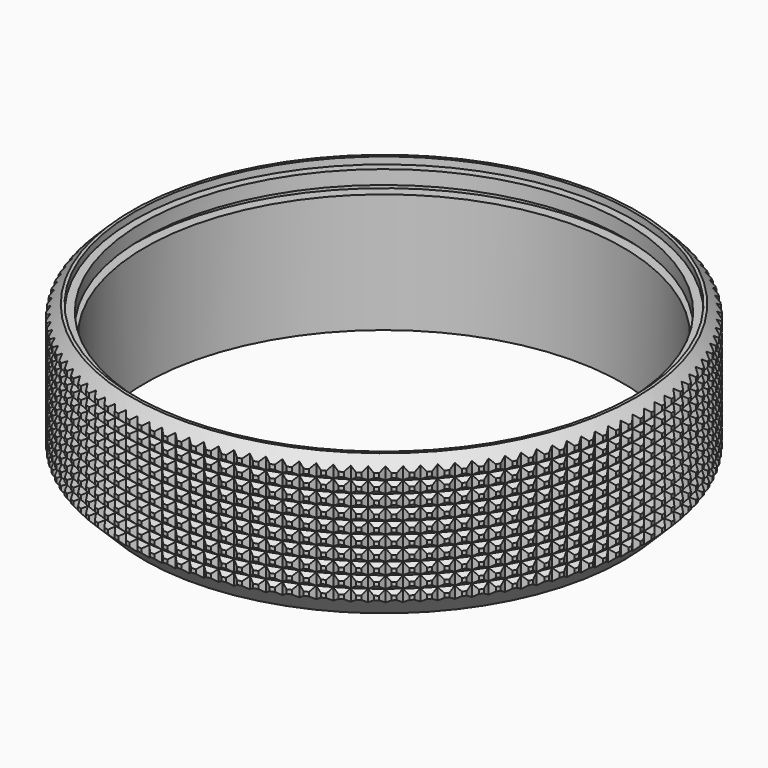
from build123d import *

# Parameters (mm, degrees)
F5_DEPTH = 14.801


# Not quite as in the source:
# - ends of sketch curves that miss each other by under 0.0002 mm in the source are joined


with BuildPart() as f1:
    # F0 (on Front) → F1 (revolve)
    with BuildSketch(Plane.XZ):
        Polygon((24, 12), (24, 0), (24.1, 0), (26.5, 2.4), (26.5, 13.65), (25.35, 14.8), (25.05, 14.8), (25.05, 14.1), (24.25, 14.1), (24.25, 12.7), (25.05, 12.7), (25.05, 12), align=None)
    revolve(axis=Axis((0, 0, 7.4), (0, 0, 1)))

    # F2 (on Front) → F3 (revolve, cut)
    with BuildSketch(Plane.XZ):
        Polygon((26.1, 3.2), (26.5, 2.8), (26.5, 3.6), align=None)
        Polygon((26.1, 4.4), (26.5, 4), (26.5, 4.8), align=None)
        Polygon((26.1, 5.6), (26.5, 5.2), (26.5, 6), align=None)
        Polygon((26.1, 6.8), (26.5, 6.4), (26.5, 7.2), align=None)
        Polygon((26.1, 8), (26.5, 7.6), (26.5, 8.4), align=None)
        Polygon((26.1, 9.2), (26.5, 8.8), (26.5, 9.6), align=None)
        Polygon((26.1, 10.4), (26.5, 10), (26.5, 10.8), align=None)
        Polygon((26.1, 11.6), (26.5, 11.2), (26.5, 12), align=None)
        Polygon((26.1, 12.8), (26.5, 12.4), (26.5, 13.2), align=None)
    revolve(axis=Axis((0, 0, 7.4), (0, 0, 1)), mode=Mode.SUBTRACT)

    # F4 (on Top) → F5 (cut, through all)
    with BuildSketch(Plane.XY):
        with BuildLine():
            ThreePointArc((19.9973857787, -17.3883455803), (24.8211676109, -9.2822216324), (26.5, 0))
            ThreePointArc((26.5, 0), (26.4989503727, 0.2358583159), (26.4958015739, 0.4716979477))
            Line((26.4958015739, 0.4716979477), (26.1022815987, 0.0027191035))
            Line((26.1022815987, 0.0027191035), (26.4942734182, -0.5174716106))
            Line((26.4942734182, -0.5174716106), (26.4834675206, -0.9174542359))
            Line((26.4834675206, -0.9174542359), (26.0659423946, -1.3651951167))
            Line((26.0659423946, -1.3651951167), (26.4301723244, -1.9051881942))
            Line((26.4301723244, -1.9051881942), (26.3984477628, -2.3040571203))
            Line((26.3984477628, -2.3040571203), (25.9580618933, -2.729332811))
            Line((25.9580618933, -2.729332811), (26.2935316046, -3.2876481685))
            Line((26.2935316046, -3.2876481685), (26.2409753337, -3.6843101233))
            Line((26.2409753337, -3.6843101233), (25.7789357878, -4.0859549729))
            Line((25.7789357878, -4.0859549729), (26.0847257813, -4.6610623066))
            Line((26.0847257813, -4.6610623066), (26.0114818543, -5.0544300673))
            Line((26.0114818543, -5.0544300673), (25.5290550502, -5.4313431951))
            Line((25.5290550502, -5.4313431951), (25.804327177, -6.021666176))
            Line((25.804327177, -6.021666176), (25.7105963503, -6.4106615489))
            Line((25.7105963503, -6.4106615489), (25.2091045865, -6.7618098623))
            Line((25.2091045865, -6.7618098623), (25.4531043446, -7.365730456))
            Line((25.4531043446, -7.365730456), (25.339143528, -7.7492872318))
            Line((25.339143528, -7.7492872318), (24.8199277527, -8.0737292567))
            Line((24.8199277527, -8.0737292567), (25.0320199616, -8.6895711598))
            Line((25.0320199616, -8.6895711598), (24.8981415136, -9.066638036))
            Line((24.8981415136, -9.066638036), (24.3626601561, -9.3634601994))
            Line((24.3626601561, -9.3634601994), (24.5422281909, -9.9895597321))
            Line((24.5422281909, -9.9895597321), (24.3887990632, -10.3591031947))
            Line((24.3887990632, -10.3591031947), (23.83848367, -10.6275099459))
            Line((23.83848367, -10.6275099459), (23.9850715178, -11.2621329946))
            Line((23.9850715178, -11.2621329946), (23.8125122489, -11.6231401506))
            Line((23.8125122489, -11.6231401506), (23.2489714437, -11.8623490302))
            Line((23.2489714437, -11.8623490302), (23.36207707, -12.5038029123))
            Line((23.36207707, -12.5038029123), (23.1708606328, -12.8552842662))
            Line((23.1708606328, -12.8552842662), (22.5955729153, -13.0646718715))
            Line((22.5955729153, -13.0646718715), (22.6749524319, -13.7111661545))
            Line((22.6749524319, -13.7111661545), (22.4656029374, -14.0521583203))
            Line((22.4656029374, -14.0521583203), (21.8801451312, -14.2311507343))
            Line((21.8801451312, -14.2311507343), (21.9255809644, -14.8809134222))
            Line((21.9255809644, -14.8809134222), (21.6986722251, -15.2104817641))
            Line((21.6986722251, -15.2104817641), (21.1046490293, -15.3585883812))
            Line((21.1046490293, -15.3585883812), (21.1160166427, -16.0098385197))
            Line((21.1160166427, -16.0098385197), (20.8721705996, -16.3270797138))
            Line((20.8721705996, -16.3270797138), (20.2712101905, -16.4438945839))
            Line((20.2712101905, -16.4438945839), (20.2484784262, -17.0948471416))
            Line((20.2484784262, -17.0948471416), (19.9973857787, -17.3883455803))
        make_face()
        with BuildLine():
            ThreePointArc((19.3254063276, -18.1322549693), (19.6602174506, -17.7686760844), (19.988189475, -17.3989161016))
            Line((19.988189475, -17.3989161016), (19.3821130127, -17.4840945935))
            Line((19.3821130127, -17.4840945935), (19.3254063276, -18.1322549693))
        make_face()
        with BuildLine():
            ThreePointArc((18.3494288956, -19.1193216199), (18.7021282663, -18.7744613321), (19.0483474604, -18.4230958046))
            Line((19.0483474604, -18.4230958046), (18.4397944495, -18.4763372942))
            Line((18.4397944495, -18.4763372942), (18.3494288956, -19.1193216199))
        make_face()
        with BuildLine():
            ThreePointArc((17.3232270711, -20.053822674), (17.6926880381, -19.72862869), (18.0560456252, -19.3966289953))
            Line((18.0560456252, -19.3966289953), (17.4468373306, -19.4179030177))
            Line((17.4468373306, -19.4179030177), (17.3232270711, -20.053822674))
        make_face()
        with BuildLine():
            ThreePointArc((16.2496342413, -20.9332125347), (16.6346788807, -20.6285592938), (17.0140130588, -20.3168245461))
            Line((17.0140130588, -20.3168245461), (16.4059632824, -20.3062109977))
            Line((16.4059632824, -20.3062109977), (16.2496342413, -20.9332125347))
        make_face()
        with BuildLine():
            ThreePointArc((15.1316119233, -21.7550987266), (15.5310163219, -21.4717845557), (15.9251174885, -21.1811386138))
            Line((15.9251174885, -21.1811386138), (15.3200252683, -21.1388264439))
            Line((15.3200252683, -21.1388264439), (15.1316119233, -21.7550987266))
        make_face()
        with BuildLine():
            ThreePointArc((13.9722414414, -22.5172482578), (14.3847411408, -22.2559929527), (14.7923572931, -21.9871818502))
            Line((14.7923572931, -21.9871818502), (14.191999769, -21.9134672152))
            Line((14.191999769, -21.9134672152), (13.9722414414, -22.5172482578))
        make_face()
        with BuildLine():
            ThreePointArc((12.7747152975, -23.2175935245), (13.1990108615, -22.9790363653), (13.6188531339, -22.7327261743))
            Line((13.6188531339, -22.7327261743), (13.0249786239, -22.628010075))
            Line((13.0249786239, -22.628010075), (12.7747152975, -23.2175935245))
        make_face()
        with BuildLine():
            ThreePointArc((11.5423282603, -23.8542377437), (11.9770909276, -23.6389359514), (12.4078392281, -23.4157110865))
            Line((12.4078392281, -23.4157110865), (11.8221605568, -23.2804965111))
            Line((11.8221605568, -23.2804965111), (11.5423282603, -23.8542377437))
        make_face()
        with BuildLine():
            ThreePointArc((10.2784681996, -24.4254599029), (10.7223455829, -24.2338875379), (11.1626542901, -24.0342495036))
            Line((11.1626542901, -24.0342495036), (10.5868424086, -23.8691381035))
            Line((10.5868424086, -23.8691381035), (10.2784681996, -24.4254599029))
        make_face()
        with BuildLine():
            ThreePointArc((8.9866066922, -24.9297192154), (9.4382284858, -24.7622665168), (9.8867321676, -24.586633097))
            Line((9.8867321676, -24.586633097), (9.3224101003, -24.3923214264))
            Line((9.3224101003, -24.3923214264), (8.9866066922, -24.9297192154))
        make_face()
        with BuildLine():
            ThreePointArc((7.6702894258, -25.3656590714), (8.1282730846, -25.222632231), (8.5835922011, -25.0713371188))
            Line((8.5835922011, -25.0713371188), (8.0323293531, -24.8486124709))
            Line((8.0323293531, -24.8486124709), (7.6702894258, -25.3656590714))
        make_face()
        with BuildLine():
            ThreePointArc((6.3331264294, -25.7321104776), (6.7960827818, -25.613731841), (7.2568293348, -25.487024699))
            Line((7.2568293348, -25.487024699), (6.7201361886, -25.2367605748))
            Line((6.7201361886, -25.2367605748), (6.3331264294, -25.7321104776))
        make_face()
        with BuildLine():
            ThreePointArc((4.9787821556, -26.0280949792), (5.4453209161, -25.9345036606), (5.9101040093, -25.8325506019))
            Line((5.9101040093, -25.8325506019), (5.389427237, -25.5557018511))
            Line((5.389427237, -25.5557018511), (4.9787821556, -26.0280949792))
        make_face()
        with BuildLine():
            ThreePointArc((3.6109654444, -26.2528270584), (4.0797005908, -26.184079955), (4.5471318666, -26.1069644307))
            Line((4.5471318666, -26.1069644307), (4.0438498791, -25.8045621041))
            Line((4.0438498791, -25.8045621041), (3.6109654444, -26.2528270584))
        make_face()
        with BuildLine():
            ThreePointArc((2.2334193938, -26.4057160064), (2.7029743789, -26.361789194), (3.1716732979, -26.3095132697))
            Line((3.1716732979, -26.3095132697), (2.6870922488, -25.982659225))
            Line((2.6870922488, -25.982659225), (2.2334193938, -26.4057160064))
        make_face()
        with BuildLine():
            ThreePointArc((0.8499111658, -26.4863672671), (1.3189239329, -26.4671577556), (1.7875228668, -26.4396437571))
            Line((1.7875228668, -26.4396437571), (1.3228731247, -26.089505062))
            Line((1.3228731247, -26.089505062), (0.8499111658, -26.4863672671))
        make_face()
        with BuildLine():
            ThreePointArc((-0.5357782445, -26.4945832515), (-0.0686504702, -26.4999110775), (0.3984986386, -26.4970035822))
            Line((0.3984986386, -26.4970035822), (-0.0450682636, -26.1248067581))
            Line((-0.0450682636, -26.1248067581), (-0.5357782445, -26.4945832515))
        make_face()
        with BuildLine():
            ThreePointArc((-1.9198642517, -26.4303636232), (-1.4559404181, -26.4599742536), (-0.9915685505, -26.4814424043))
            Line((-0.9915685505, -26.4814424043), (-1.4129824838, -26.0884675538))
            Line((-1.4129824838, -26.0884675538), (-1.9198642517, -26.4303636232))
        make_face()
        with BuildLine():
            ThreePointArc((-3.2985689057, -26.2939050575), (-2.8391398596, -26.3474720772), (-2.3788458534, -26.3930121889))
            Line((-2.3788458534, -26.3930121889), (-2.7771201782, -25.9805870524))
            Line((-2.7771201782, -25.9805870524), (-3.2985689057, -26.2939050575))
        make_face()
        with BuildLine():
            ThreePointArc((-4.6681310752, -26.0856004774), (-4.2144555765, -26.1627285311), (-3.7595091685, -26.2319669642))
            Line((-3.7595091685, -26.2319669642), (-4.13374234, -25.8014609467))
            Line((-4.13374234, -25.8014609467), (-4.6681310752, -26.0856004774))
        make_face()
        with BuildLine():
            ThreePointArc((-6.0248165627, -25.80603777), (-5.5781176021, -25.9062657289), (-5.1297538595, -25.9987619963))
            Line((-5.1297538595, -25.9987619963), (-5.4791305622, -25.5515802091))
            Line((-5.4791305622, -25.5515802091), (-6.0248165627, -25.80603777))
        make_face()
        with BuildLine():
            ThreePointArc((-7.3649281249, -25.4559979909), (-6.926389559, -25.5788023112), (-6.4858054077, -25.6940523899))
            Line((-6.4858054077, -25.6940523899), (-6.8095972293, -25.2316297452))
            Line((-6.8095972293, -25.2316297452), (-7.3649281249, -25.4559979909))
        make_face()
        with BuildLine():
            ThreePointArc((-8.6848153742, -25.0364530618), (-8.2555788861, -25.1812513044), (-7.8239299645, -25.3186911177))
            Line((-7.8239299645, -25.3186911177), (-8.1214956246, -24.842486517))
            Line((-8.1214956246, -24.842486517), (-8.6848153742, -25.0364530618))
        make_face()
        with BuildLine():
            ThreePointArc((-9.9808845358, -24.5485629698), (-9.5620469282, -24.7147174482), (-9.1404447724, -24.8737264873))
            Line((-9.1404447724, -24.8737264873), (-9.4112299258, -24.385217139))
            Line((-9.4112299258, -24.385217139), (-9.9808845358, -24.5485629698))
        make_face()
        with BuildLine():
            ThreePointArc((-11.2496080368, -23.9936724788), (-10.8422188593, -24.1804940025), (-10.4317284256, -24.3603990537))
            Line((-10.4317284256, -24.3603990537), (-10.6752650608, -23.8610749549))
            Line((-10.6752650608, -23.8610749549), (-11.2496080368, -23.9936724788))
        make_face()
        with BuildLine():
            ThreePointArc((-12.4875339043, -23.373307361), (-12.0925934154, -23.5800590434), (-11.6942309379, -23.7801379889))
            Line((-11.6942309379, -23.7801379889), (-11.9101363971, -23.2714966019))
            Line((-11.9101363971, -23.2714966019), (-12.4875339043, -23.373307361))
        make_face()
        with BuildLine():
            ThreePointArc((-13.6912949486, -22.6891701618), (-13.3097524077, -22.9150712599), (-12.9244835908, -23.1345569206))
            Line((-12.9244835908, -23.1345569206), (-13.1124592383, -22.6180980734))
            Line((-13.1124592383, -22.6180980734), (-13.6912949486, -22.6891701618))
        make_face()
        with BuildLine():
            ThreePointArc((-14.8576177102, -21.9431355093), (-14.490369994, -22.1873652658), (-14.1191085318, -22.4254492545))
            Line((-14.1191085318, -22.4254492545), (-14.278938101, -21.9026702891))
            Line((-14.278938101, -21.9026702891), (-14.8576177102, -21.9431355093))
        make_face()
        with BuildLine():
            ThreePointArc((-15.9833311488, -21.137244981), (-15.6312216817, -21.3989464399), (-15.2748280974, -21.6547829958))
            Line((-15.2748280974, -21.6547829958), (-15.4063757478, -21.1271741871))
            Line((-15.4063757478, -21.1271741871), (-15.9833311488, -21.137244981))
        make_face()
        with BuildLine():
            ThreePointArc((-17.0653750537, -20.2737015435), (-16.7291930408, -20.5519853105), (-16.3884738325, -20.8246950864))
            Line((-16.3884738325, -20.8246950864), (-16.4916819504, -20.2937353482))
            Line((-16.4916819504, -20.2937353482), (-17.0653750537, -20.2737015435))
        make_face()
        with BuildLine():
            ThreePointArc((-18.1008081556, -19.3548635778), (-17.7812881023, -19.6488115016), (-17.4569951829, -19.9374852773))
            Line((-17.4569951829, -19.9374852773), (-17.53188196, -19.4046381703))
            Line((-17.53188196, -19.4046381703), (-18.1008081556, -19.3548635778))
        make_face()
        with BuildLine():
            ThreePointArc((-19.0868159201, -18.3832385077), (-18.7846374227, -18.6919072569), (-18.4774678359, -18.9956095552))
            Line((-18.4774678359, -18.9956095552), (-18.5241246606, -18.4623196071))
            Line((-18.5241246606, -18.4623196071), (-19.0868159201, -18.3832385077))
        make_face()
        with BuildLine():
            ThreePointArc((-20.0207180056, -17.3614760473), (-19.7365057923, -17.6839005627), (-19.4471016863, -18.0016731445))
            Line((-19.4471016863, -18.0016731445), (-19.465690384, -17.4693624881))
            Line((-19.465690384, -17.4693624881), (-20.0207180056, -17.3614760473))
        make_face()
        with BuildLine():
            ThreePointArc((-20.8999753661, -16.2923610841), (-20.6342995693, -16.627557887), (-20.363248408, -16.9584231069))
            Line((-20.363248408, -16.9584231069), (-20.3539983639, -16.4284884398))
            Line((-20.3539983639, -16.4284884398), (-20.8999753661, -16.2923610841))
        make_face()
        with BuildLine():
            ThreePointArc((-21.7221969847, -15.1788062166), (-21.4755736198, -15.5257765571), (-21.2234086088, -15.868740562))
            Line((-21.2234086088, -15.868740562), (-21.18661381, -15.3425504256))
            Line((-21.18661381, -15.3425504256), (-21.7221969847, -15.1788062166))
        make_face()
        with BuildLine():
            ThreePointArc((-22.4851462186, -14.0238439641), (-22.2580378484, -14.381576796), (-22.0252385523, -14.7356325522))
            Line((-22.0252385523, -14.7356325522), (-21.9612545812, -14.2145249262))
            Line((-21.9612545812, -14.2145249262), (-22.4851462186, -14.0238439641))
        make_face()
        with BuildLine():
            ThreePointArc((-23.1867467437, -12.8306186695), (-22.979563302, -13.19809344), (-22.7665564287, -13.562223578))
            Line((-22.7665564287, -13.562223578), (-22.6757974409, -13.0475037811))
            Line((-22.6757974409, -13.0475037811), (-23.1867467437, -12.8306186695))
        make_face()
        with BuildLine():
            ThreePointArc((-23.8250880823, -11.6023781127), (-23.638187832, -11.9785673609), (-23.4453481591, -12.3517468278))
            Line((-23.4453481591, -12.3517468278), (-23.3282838768, -11.844685714))
            Line((-23.3282838768, -11.844685714), (-23.8250880823, -11.6023781127))
        make_face()
        with BuildLine():
            ThreePointArc((-24.3984307012, -10.3424648571), (-24.2321213026, -10.7263366148), (-24.0597727197, -11.1075351305))
            Line((-24.0597727197, -11.1075351305), (-23.9169254691, -10.6093675657))
            Line((-23.9169254691, -10.6093675657), (-24.3984307012, -10.3424648571))
        make_face()
        with BuildLine():
            ThreePointArc((-24.9052106681, -9.0543073493), (-24.7597503312, -9.4448273428), (-24.6081669733, -9.8330116554))
            Line((-24.6081669733, -9.8330116554), (-24.440108792, -9.3449352574))
            Line((-24.440108792, -9.3449352574), (-24.9052106681, -9.0543073493))
        make_face()
        with BuildLine():
            ThreePointArc((-25.344043855, -7.7414107936), (-25.2196425504, -8.1375444471), (-25.0890499967, -8.5316803892))
            Line((-25.0890499967, -8.5316803892), (-24.8963998363, -8.0548545101))
            Line((-24.8963998363, -8.0548545101), (-25.344043855, -7.7414107936))
        make_face()
        with BuildLine():
            ThreePointArc((-25.7137296763, -6.4073478237), (-25.6105503823, -6.8080620675), (-25.5011268961, -7.2071164155))
            Line((-25.5011268961, -7.2071164155), (-25.28454794, -6.7426613455))
            Line((-25.28454794, -6.7426613455), (-25.7137296763, -6.4073478237))
        make_face()
        with BuildLine():
            ThreePointArc((-26.2417937031, -3.6902931106), (-26.1813656761, -4.0970832717), (-26.114632133, -4.5028866918))
            Line((-26.114632133, -4.5028866918), (-25.8523494691, -4.0663750359))
            Line((-25.8523494691, -4.0663750359), (-26.2417937031, -3.6902931106))
        make_face()
        with BuildLine():
            ThreePointArc((-26.3987154191, -2.3146974362), (-26.3597288935, -2.7229933279), (-26.3144278386, -3.1306369207))
            Line((-26.3144278386, -3.1306369207), (-26.0304465899, -2.7096174057))
            Line((-26.0304465899, -2.7096174057), (-26.3987154191, -2.3146974362))
        make_face()
        with BuildLine():
            ThreePointArc((-26.4835808797, -0.9327077735), (-26.4660232432, -1.3414968095), (-26.4421560938, -1.749966032))
            Line((-26.4421560938, -1.749966032), (-26.1372924267, -1.3453982815))
            Line((-26.1372924267, -1.3453982815), (-26.4835808797, -0.9327077735))
        make_face()
        with BuildLine():
            ThreePointArc((-26.4961464362, 0.4519115291), (-26.4999640768, 0.0436340064), (-26.4974909671, -0.3646538746))
            Line((-26.4974909671, -0.3646538746), (-26.1725941227, 0.0225431068))
            Line((-26.1725941227, 0.0225431068), (-26.4961464362, 0.4519115291))
        make_face()
        with BuildLine():
            ThreePointArc((-26.436364202, 1.8353876375), (-26.4614635277, 1.4286175046), (-26.4803043482, 1.0215094838))
            Line((-26.4803043482, 1.0215094838), (-26.1362549183, 1.390457327))
            Line((-26.1362549183, 1.390457327), (-26.436364202, 1.8353876375))
        make_face()
        with BuildLine():
            ThreePointArc((-26.3043823292, 3.2139493272), (-26.3506306947, 2.8096729331), (-26.3906660406, 2.4047340671))
            Line((-26.3906660406, 2.4047340671), (-26.0283744167, 2.7545950213))
            Line((-26.0283744167, 2.7545950213), (-26.3043823292, 3.2139493272))
        make_face()
        with BuildLine():
            ThreePointArc((-26.1005447742, 4.5838370924), (-26.1677713042, 4.1830305962), (-26.2288433215, 3.7812402748))
            Line((-26.2288433215, 3.7812402748), (-25.849248311, 4.1112171831))
            Line((-25.849248311, 4.1112171831), (-26.1005447742, 4.5838370924))
        make_face()
        with BuildLine():
            ThreePointArc((-26.0132543546, -5.0557489934), (-25.9314143151, -5.4600138844), (-25.8432921014, -5.8629560261))
            Line((-25.8432921014, -5.8629560261), (-25.6034892163, -5.4119523939))
            Line((-25.6034892163, -5.4119523939), (-26.0132543546, -5.0557489934))
        make_face()
        with BuildLine():
            ThreePointArc((-25.8253905485, 5.9413132403), (-25.9133868502, 5.5449420151), (-25.995299973, 5.1472691124))
            Line((-25.995299973, 5.1472691124), (-25.5993675732, 5.4566054053))
            Line((-25.5993675732, 5.4566054053), (-25.8253905485, 5.9413132403))
        make_face()
        with BuildLine():
            ThreePointArc((-25.4796524563, 7.2826719481), (-25.5881732165, 6.8916900282), (-25.6906947891, 6.4990923407))
            Line((-25.6906947891, 6.4990923407), (-25.2794171091, 6.7870720724))
            Line((-25.2794171091, 6.7870720724), (-25.4796524563, 7.2826719481))
        make_face()
        with BuildLine():
            ThreePointArc((-25.0642553199, 8.6042492559), (-25.1930187842, 8.2195988065), (-25.3158795664, 7.8330225189))
            Line((-25.3158795664, 7.8330225189), (-24.8902738808, 8.0989704676))
            Line((-24.8902738808, 8.0989704676), (-25.0642553199, 8.6042492559))
        make_face()
        with BuildLine():
            Line((-24.4330045027, 9.3887047688), (-24.5803136937, 9.9024329696))
            ThreePointArc((-24.5803136937, 9.9024329696), (-24.72900203, 9.5250437585), (-24.8718965842, 9.1454229155))
            Line((-24.8718965842, 9.1454229155), (-24.4330045027, 9.3887047688))
        make_face()
        with BuildLine():
            Line((-23.9088623185, 10.6527399037), (-24.0291290729, 11.1736724491))
            ThreePointArc((-24.0291290729, 11.1736724491), (-24.1973886206, 10.8044612982), (-24.3599755854, 10.4327172624))
            Line((-24.3599755854, 10.4327172624), (-23.9088623185, 10.6527399037))
        make_face()
        with BuildLine():
            Line((-23.3192839654, 11.88761124), (-23.4121865988, 12.4144882562))
            ThreePointArc((-23.4121865988, 12.4144882562), (-23.5996280113, 12.0543584535), (-23.7815302658, 11.6913993267))
            Line((-23.7815302658, 11.6913993267), (-23.3192839654, 11.88761124))
        make_face()
        with BuildLine():
            Line((-22.6658854367, 13.0899340811), (-22.7311512697, 13.6214816358))
            ThreePointArc((-22.7311512697, 13.6214816358), (-22.937349558, 13.2713222874), (-23.1381542847, 12.918042278))
            Line((-23.1381542847, 12.918042278), (-22.6658854367, 13.0899340811))
        make_face()
        with BuildLine():
            Line((-21.9504576524, 14.2564129438), (-21.9878636621, 14.7913438057))
            ThreePointArc((-21.9878636621, 14.7913438057), (-22.21235815, 14.4520291107), (-22.4316168083, 14.1093078273))
            Line((-22.4316168083, 14.1093078273), (-21.9504576524, 14.2564129438))
        make_face()
        with BuildLine():
            Line((-21.1749615503, 15.3838505905), (-21.1843351721, 15.9208650304))
            ThreePointArc((-21.1843351721, 15.9208650304), (-21.426629378, 15.593253461), (-21.6638575988, 15.2619551153))
            Line((-21.6638575988, 15.2619551153), (-21.1749615503, 15.3838505905))
        make_face()
        with BuildLine():
            Line((-20.3415227113, 16.469156793), (-20.3227427872, 17.0069434528))
            ThreePointArc((-20.3227427872, 17.0069434528), (-20.5823042456, 16.691876825), (-20.8369816638, 16.3728493288))
            Line((-20.8369816638, 16.3728493288), (-20.3415227113, 16.469156793))
        make_face()
        with BuildLine():
            Line((-19.4524255333, 17.5093568025), (-19.4054233985, 18.0465936599))
            ThreePointArc((-19.4054233985, 18.0465936599), (-19.6816834403, 17.7448960818), (-19.9532534809, 17.4389700248))
            Line((-19.9532534809, 17.4389700248), (-19.4524255333, 17.5093568025))
        make_face()
        with BuildLine():
            Line((-18.5101069699, 18.501599503), (-18.4348676672, 19.0369549585))
            ThreePointArc((-18.4348676672, 19.0369549585), (-18.7272211763, 18.7494316451), (-19.0150908131, 18.4574191416))
            Line((-19.0150908131, 18.4574191416), (-18.5101069699, 18.501599503))
        make_face()
        with BuildLine():
            Line((-17.5171498508, 19.4431652263), (-17.4137134577, 19.9752993373))
            ThreePointArc((-17.4137134577, 19.9752993373), (-17.7215186251, 19.7027352827), (-18.0250581319, 19.4254286784))
            Line((-18.0250581319, 19.4254286784), (-17.5171498508, 19.4431652263))
        make_face()
        with BuildLine():
            Line((-16.4762758024, 20.3314732062), (-16.3447388539, 20.859039091))
            ThreePointArc((-16.3447388539, 20.859039091), (-16.6673169507, 20.6021975931), (-16.9858596656, 20.3403680257))
            Line((-16.9858596656, 20.3403680257), (-16.4762758024, 20.3314732062))
        make_face()
        with BuildLine():
            Line((-15.3903377882, 21.1640886521), (-15.2308547741, 21.685734086))
            ThreePointArc((-15.2308547741, 21.685734086), (-15.567489965, 21.4453551192), (-15.9003320907, 21.1997509279))
            Line((-15.9003320907, 21.1997509279), (-15.3903377882, 21.1640886521))
        make_face()
        with BuildLine():
            Line((-14.2623122887, 21.9387294232), (-14.0750972026, 22.4530986444))
            ThreePointArc((-14.0750972026, 22.4530986444), (-14.4250364235, 22.2298970798), (-14.7714368857, 22.0012420634))
            Line((-14.7714368857, 22.0012420634), (-14.2623122887, 21.9387294232))
        make_face()
        with BuildLine():
            Line((-13.0952911435, 22.6532722828), (-12.8806190571, 23.1590080251))
            ThreePointArc((-12.8806190571, 23.1590080251), (-13.2430719797, 22.9536717006), (-13.6022523667, 22.7426632247))
            Line((-13.6022523667, 22.7426632247), (-13.0952911435, 22.6532722828))
        make_face()
        with BuildLine():
            Line((-11.8924730764, 23.3057587186), (-11.6506817112, 23.8015044832))
            ThreePointArc((-11.6506817112, 23.8015044832), (-12.0248208178, 23.614692128), (-12.3959654242, 23.4219990864))
            Line((-12.3959654242, 23.4219990864), (-11.8924730764, 23.3057587186))
        make_face()
        with BuildLine():
            Line((-10.657154928, 23.8944003108), (-10.3886461949, 24.3788028877))
            ThreePointArc((-10.3886461949, 24.3788028877), (-10.7736069857, 24.2111419086), (-11.1558629835, 24.0374025447))
            Line((-11.1558629835, 24.0374025447), (-10.657154928, 23.8944003108))
        make_face()
        with BuildLine():
            Line((-9.3927226197, 24.4175836335), (-9.0979640946, 24.8892958786))
            ThreePointArc((-9.0979640946, 24.8892958786), (-9.49284545, 24.7413800193), (-9.8853232078, 24.5871996185))
            Line((-9.8853232078, 24.5871996185), (-9.3927226197, 24.4175836335))
        make_face()
        with BuildLine():
            Line((-8.1026418723, 24.8738746777), (-7.7821681759, 25.3315585482))
            ThreePointArc((-7.7821681759, 25.3315585482), (-8.1860328949, 25.2039454341), (-8.5878064678, 25.0698938983))
            Line((-8.5878064678, 25.0698938983), (-8.1026418723, 24.8738746777))
        make_face()
        with BuildLine():
            Line((-6.7904487077, 25.2620227813), (-6.4448627556, 25.7043526287))
            ThreePointArc((-6.4448627556, 25.7043526287), (-6.8567382892, 25.5975612126), (-7.266846099, 25.4841705334))
            Line((-7.266846099, 25.4841705334), (-6.7904487077, 25.2620227813))
        make_face()
        with BuildLine():
            Line((-5.4597397561, 25.5809640574), (-5.0897138468, 26.006630173))
            ThreePointArc((-5.0897138468, 26.006630173), (-5.508593246, 25.921138101), (-5.9260389688, 25.828899747))
            Line((-5.9260389688, 25.828899747), (-5.4597397561, 25.5809640574))
        make_face()
        with BuildLine():
            Line((-4.1141623981, 25.8298243101), (-3.7204391053, 26.2375367149))
            ThreePointArc((-3.7204391053, 26.2375367149), (-4.1452821984, 26.1737776314), (-4.5690358785, 26.1031398713))
            Line((-4.5690358785, 26.1031398713), (-4.1141623981, 25.8298243101))
        make_face()
        with BuildLine():
            Line((-2.7574047678, 26.0079214308), (-2.3407976036, 26.3964138962))
            ThreePointArc((-2.3407976036, 26.3964138962), (-2.7705324187, 26.3547747119), (-3.1995318213, 26.306139894))
            Line((-3.1995318213, 26.306139894), (-2.7574047678, 26.0079214308))
        make_face()
        with BuildLine():
            Line((-1.3931856437, 26.1147672675), (-0.9545794625, 26.4828015521))
            ThreePointArc((-0.9545794625, 26.4828015521), (-1.3881039053, 26.4636196985), (-1.821256122, 26.4373415104))
            Line((-1.821256122, 26.4373415104), (-1.3931856437, 26.1147672675))
        make_face()
        with BuildLine():
            Line((-0.0252442553, 26.1500689634), (0.4344046323, 26.4964392441))
            ThreePointArc((0.4344046323, 26.4964392441), (-0.0017791655, 26.4999999403), (-0.4379624814, 26.4963806748))
            Line((-0.4379624814, 26.4963806748), (-0.0252442553, 26.1500689634))
        make_face()
        with BuildLine():
            Line((1.3426699649, 26.1137297588), (1.8223339977, 26.437267234))
            ThreePointArc((1.8223339977, 26.437267234), (1.3846470799, 26.463800794), (0.94658105, 26.4830886476))
            Line((0.94658105, 26.4830886476), (1.3426699649, 26.1137297588))
        make_face()
        with BuildLine():
            Line((2.7068076592, 26.0058492571), (3.2053885743, 26.3054268942))
            ThreePointArc((3.2053885743, 26.3054268942), (2.7673782425, 26.3551061023), (2.3286021436, 26.3974925335))
            Line((2.3286021436, 26.3974925335), (2.7068076592, 26.0058492571))
        make_face()
        with BuildLine():
            Line((4.0634298209, 25.8267231512), (4.5797595717, 26.1012605494))
            ThreePointArc((4.5797595717, 26.1012605494), (4.1426262343, 26.1741981326), (3.7043342861, 26.2398153099))
            Line((3.7043342861, 26.2398153099), (4.0634298209, 25.8267231512))
        make_face()
        with BuildLine():
            Line((5.4088180431, 25.5768424133), (5.9416601053, 25.8253107473))
            ThreePointArc((5.9416601053, 25.8253107473), (5.5066218304, 25.9215569752), (5.0700268684, 26.0104753427))
            Line((5.0700268684, 26.0104753427), (5.4088180431, 25.5768424133))
        make_face()
        with BuildLine():
            Line((6.7392847102, 25.2568919491), (7.2873357941, 25.4783189599))
            ThreePointArc((7.2873357941, 25.4783189599), (6.8556249989, 25.5978594002), (6.421955246, 25.7100853911))
            Line((6.421955246, 25.7100853911), (6.7392847102, 25.2568919491))
        make_face()
        with BuildLine():
            Line((8.0511831054, 24.8677487207), (8.6130752882, 25.0612237147))
            ThreePointArc((8.6130752882, 25.0612237147), (8.1859351672, 25.203977175), (7.7564307449, 25.339451101))
            Line((7.7564307449, 25.339451101), (8.0511831054, 24.8677487207))
        make_face()
        with BuildLine():
            Line((9.3409174065, 24.4104793425), (9.915220694, 24.57515816))
            ThreePointArc((9.915220694, 24.57515816), (9.4939013999, 24.7409748435), (9.069810588, 24.8995689902))
            Line((9.069810588, 24.8995689902), (9.3409174065, 24.4104793425))
        make_face()
        with BuildLine():
            Line((10.6049525414, 23.8863371581), (11.1901778657, 24.02144707))
            ThreePointArc((11.1901778657, 24.02144707), (10.7759324567, 24.2101069739), (10.358507717, 24.3916239287))
            Line((10.358507717, 24.3916239287), (10.6049525414, 23.8863371581))
        make_face()
        with BuildLine():
            Line((11.8398238776, 23.2967588049), (12.4344265326, 23.4016032956))
            ThreePointArc((12.4344265326, 23.4016032956), (12.0285067046, 23.6128148779), (11.6190004848, 23.8169861178))
            Line((11.6190004848, 23.8169861178), (11.8398238776, 23.2967588049))
        make_face()
        with BuildLine():
            Line((13.0421467187, 22.6433602761), (13.6445302311, 22.717323671))
            ThreePointArc((13.6445302311, 22.717323671), (13.2481818547, 22.9507228109), (12.8478421922, 23.1772075756))
            Line((12.8478421922, 23.1772075756), (13.0421467187, 22.6433602761))
        make_face()
        with BuildLine():
            Line((14.2086255813, 21.9279324917), (14.8171460101, 21.9704843851))
            ThreePointArc((14.8171460101, 21.9704843851), (14.4316044974, 22.2256336609), (14.0416704459, 22.474018134))
            Line((14.0416704459, 22.474018134), (14.2086255813, 21.9279324917))
        make_face()
        with BuildLine():
            Line((15.3360632279, 21.1524363895), (15.9490338818, 21.1631358318))
            ThreePointArc((15.9490338818, 21.1631358318), (15.5755194077, 21.4395241361), (15.1972163112, 21.7093209565))
            Line((15.1972163112, 21.7093209565), (15.3360632279, 21.1524363895))
        make_face()
        with BuildLine():
            Line((16.4213694304, 20.3189975503), (17.0370659874, 20.2974969526))
            ThreePointArc((17.0370659874, 20.2974969526), (16.6767785943, 20.5945394636), (16.3113132364, 20.8851875861))
            Line((16.3113132364, 20.8851875861), (16.4213694304, 20.3189975503))
        make_face()
        with BuildLine():
            Line((17.4615694398, 19.4299003723), (18.0782354498, 19.375949087))
            ThreePointArc((18.0782354498, 19.375949087), (17.7323500665, 19.6929876128), (17.380905724, 20.0038525343))
            Line((17.380905724, 20.0038525343), (17.4615694398, 19.4299003723))
        make_face()
        with BuildLine():
            Line((18.4538121402, 18.4875818088), (19.0696648863, 18.4010293496))
            ThreePointArc((19.0696648863, 18.4010293496), (18.7393262927, 18.7373330572), (18.4030577258, 19.0677074223))
            Line((18.4030577258, 19.0677074223), (18.4538121402, 18.4875818088))
        make_face()
        with BuildLine():
            Line((19.3953778634, 17.4946246896), (20.0086145547, 17.3754235518))
            ThreePointArc((20.0086145547, 17.3754235518), (19.6949323263, 17.7301900909), (19.3749607373, 18.0792946883))
            Line((19.3749607373, 18.0792946883), (19.3953778634, 17.4946246896))
        make_face()
        with BuildLine():
            Line((20.2836858431, 16.4537506411), (20.8924901073, 16.3019586896))
            ThreePointArc((20.8924901073, 16.3019586896), (20.5965335751, 16.6743157188), (20.2939415708, 17.0413008753))
            Line((20.2939415708, 17.0413008753), (20.2836858431, 16.4537506411))
        make_face()
        with BuildLine():
            Line((21.116301289, 15.3678126268), (21.7188499296, 15.1835950201))
            ThreePointArc((21.7188499296, 15.1835950201), (21.4416431899, 15.572602137), (21.1574697828, 15.956549514))
            Line((21.1574697828, 15.956549514), (21.116301289, 15.3678126268))
        make_face()
        with BuildLine():
            Line((21.8909420599, 14.2397871273), (22.4854120407, 14.0234177489))
            ThreePointArc((22.4854120407, 14.0234177489), (22.2279290522, 14.428068826), (21.963164736, 14.8279936195))
            Line((21.963164736, 14.8279936195), (21.8909420599, 14.2397871273))
        make_face()
        with BuildLine():
            Line((22.6054849194, 13.072765982), (23.1900605335, 12.8246283554))
            ThreePointArc((23.1900605335, 12.8246283554), (22.9532203384, 13.2438542765), (22.7088022744, 13.6587078181))
            Line((22.7088022744, 13.6587078181), (22.6054849194, 13.072765982))
        make_face()
        with BuildLine():
            Line((23.2579713551, 11.8699479148), (23.8308515364, 11.5905355808))
            ThreePointArc((23.8308515364, 11.5905355808), (23.6155136407, 12.023207371), (23.3923209918, 12.4518801238))
            Line((23.3923209918, 12.4518801238), (23.2579713551, 11.8699479148))
        make_face()
        with BuildLine():
            Line((23.8466129472, 10.6346297664), (24.4060186778, 10.3245461062))
            ThreePointArc((24.4060186778, 10.3245461062), (24.2129786274, 10.7694784455), (24.011828074, 11.2108033853))
            Line((24.011828074, 11.2108033853), (23.8466129472, 10.6346297664))
        make_face()
        with BuildLine():
            Line((24.3697962698, 9.370197458), (24.913978036, 9.0301549501))
            ThreePointArc((24.913978036, 9.0301549501), (24.7439632238, 9.4861100551), (24.5656046982, 9.938866425))
            Line((24.5656046982, 9.938866425), (24.3697962698, 9.370197458))
        make_face()
        with BuildLine():
            Line((24.8260873138, 8.0801167106), (25.3533325613, 7.7109356136))
            ThreePointArc((25.3533325613, 7.7109356136), (25.2069982982, 8.1766274707), (25.0521109704, 8.639544891))
            Line((25.0521109704, 8.639544891), (24.8260873138, 8.0801167106))
        make_face()
        with BuildLine():
            Line((25.2142354174, 6.7679235459), (25.7228759566, 6.3705300033))
            ThreePointArc((25.7228759566, 6.3705300033), (25.6008018386, 6.8446289322), (25.4699903872, 7.3163918482))
            Line((25.4699903872, 7.3163918482), (25.2142354174, 6.7679235459))
        make_face()
        with BuildLine():
            Line((25.5331766933, 5.4372145943), (26.0215960048, 5.012638164))
            ThreePointArc((26.0215960048, 5.012638164), (25.9242826072, 5.4937756873), (25.8180738042, 5.97302813))
            Line((25.8180738042, 5.97302813), (25.5331766933, 5.4372145943))
        make_face()
        with BuildLine():
            Line((25.7820369459, 4.0916372363), (26.2486773349, 3.6410078504))
            ThreePointArc((26.2486773349, 3.6410078504), (26.1765432603, 4.1277818427), (26.0953829006, 4.6131324792))
            Line((26.0953829006, 4.6131324792), (25.7820369459, 4.0916372363))
        make_face()
        with BuildLine():
            Line((25.9601340664, 2.734879606), (26.4035036182, 2.2594239713))
            ThreePointArc((26.4035036182, 2.2594239713), (26.3568829249, 2.7504040582), (26.3011331255, 3.240431501))
            Line((26.3011331255, 3.240431501), (25.9601340664, 2.734879606))
        make_face()
        with BuildLine():
            Line((26.0669799067, 1.3706604868), (26.4856591892, 0.8716979477))
            ThreePointArc((26.4856591892, 0.8716979477), (26.464799222, 1.3654311177), (26.4347361155, 1.8586894588))
            Line((26.4347361155, 1.8586894588), (26.0669799067, 1.3706604868))
        make_face()
    extrude(amount=F5_DEPTH, mode=Mode.SUBTRACT)


solid = f1.part
